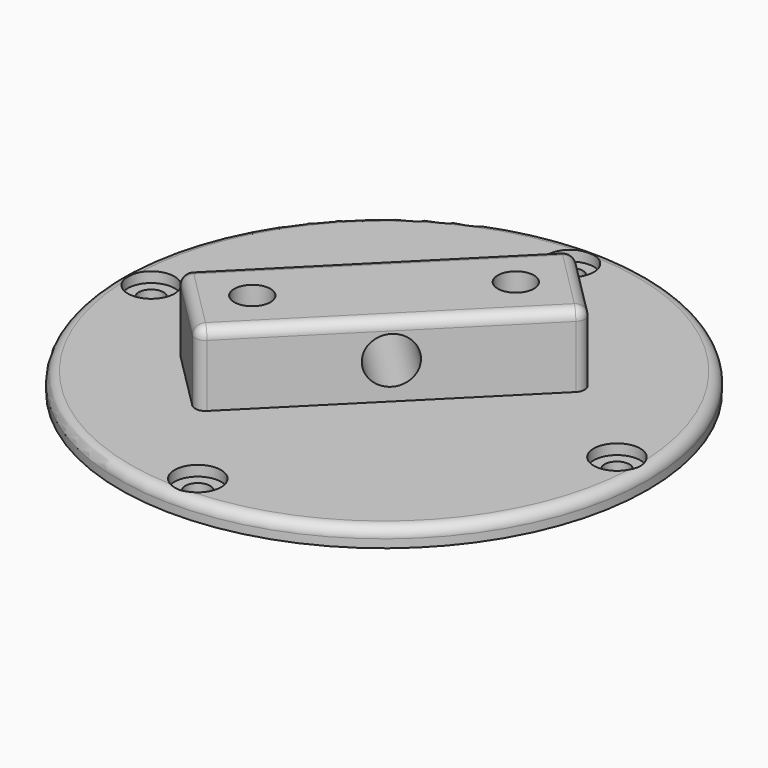
from build123d import *

# Parameters (mm, degrees)
F0_R         = 25.5
F0_R_2       = 1.2
F1_DEPTH     = 1.8
F2_R         = 2.25
F3_DEPTH     = 1
F4_R         = 1.75
F5_DEPTH     = 7
F6_START     = 2
F6_DEPTH     = 3
F7_R         = 2.25
F8_DEPTH     = 41.0634458405
F9_T1_DEPTH  = 6
F9_T3_DEPTH  = 8
F9_T5_DEPTH  = 28
F9_T7_DEPTH  = 28
F9_T9_DEPTH  = 8
F9_S13_W     = 1
F9_S13_H     = 1
F9_T14_DEPTH = 1
F9_T20_DEPTH = 1
F9_S25_W     = 1
F9_S25_H     = 1
F9_T26_DEPTH = 1
F9_T32_DEPTH = 1


# Not quite as in the source:
# - a fillet or chamfer that OpenCascade refuses, or shapes differently, is made with other operations: its cross-section is extruded or revolved along the edge and cut away or added


with BuildPart() as f1:
    # F0 (on Top) → F1 (new body)
    with BuildSketch(Plane.XY):
        Circle(F0_R)
        with Locations((0, -22.5)):
            Circle(F0_R_2, mode=Mode.SUBTRACT)
        with Locations((-22.5, 0)):
            Circle(F0_R_2, mode=Mode.SUBTRACT)
        with Locations((22.5, 0)):
            Circle(F0_R_2, mode=Mode.SUBTRACT)
        with Locations((0, 22.5)):
            Circle(F0_R_2, mode=Mode.SUBTRACT)
    extrude(amount=F1_DEPTH)

    # F2 (on face) → F3 (cut)
    with BuildSketch(Plane.XY.offset(1.8)):
        with Locations((0, -22.5)):
            Circle(F2_R)
        with Locations((-22.5, 0)):
            Circle(F2_R)
        with Locations((0, 22.5)):
            Circle(F2_R)
        with Locations((22.5, 0)):
            Circle(F2_R)
    extrude(amount=-F3_DEPTH, mode=Mode.SUBTRACT)

    # F4 (on face) → F5 (join)
    with BuildSketch(Plane.XY.offset(1.8)):
        Polygon((7.0710678119, 14.1421356237), (-14.1421356237, -7.0710678119), (-7.0710678119, -14.1421356237), (14.1421356237, 7.0710678119), align=None)
        Polygon((-6.1744923397, -10.4171330268), (-9.5205575546, -9.5205575546), (-10.4171330268, -6.1744923397), (-7.967643284, -3.7250025969), (-4.6215780691, -4.6215780691), (-3.7250025969, -7.967643284), align=None, mode=Mode.SUBTRACT)
        Polygon((3.7250025969, 7.967643284), (6.1744923397, 10.4171330268), (9.5205575546, 9.5205575546), (10.4171330268, 6.1744923397), (7.967643284, 3.7250025969), (4.6215780691, 4.6215780691), align=None, mode=Mode.SUBTRACT)
        Polygon((-10.4171330268, -6.1744923397), (-9.5205575546, -9.5205575546), (-6.1744923397, -10.4171330268), (-3.7250025969, -7.967643284), (-4.6215780691, -4.6215780691), (-7.967643284, -3.7250025969), align=None)
        with Locations((-7.0710678119, -7.0710678119)):
            Circle(F4_R, mode=Mode.SUBTRACT)
        Polygon((9.5205575546, 9.5205575546), (6.1744923397, 10.4171330268), (3.7250025969, 7.967643284), (4.6215780691, 4.6215780691), (7.967643284, 3.7250025969), (10.4171330268, 6.1744923397), align=None)
        with Locations((7.0710678119, 7.0710678119)):
            Circle(F4_R, mode=Mode.SUBTRACT)
    extrude(amount=F5_DEPTH)

    # F4 (on face) → F6 (cut)
    with BuildSketch(Plane.XY.offset(1.8).offset(F6_START)):
        Polygon((-10.4171330268, -6.1744923397), (-9.5205575546, -9.5205575546), (-6.1744923397, -10.4171330268), (-3.7250025969, -7.967643284), (-4.6215780691, -4.6215780691), (-7.967643284, -3.7250025969), align=None)
        with Locations((-7.0710678119, -7.0710678119)):
            Circle(F4_R, mode=Mode.SUBTRACT)
        Polygon((9.5205575546, 9.5205575546), (6.1744923397, 10.4171330268), (3.7250025969, 7.967643284), (4.6215780691, 4.6215780691), (7.967643284, 3.7250025969), (10.4171330268, 6.1744923397), align=None)
        with Locations((7.0710678119, 7.0710678119)):
            Circle(F4_R, mode=Mode.SUBTRACT)
    extrude(amount=F6_DEPTH, mode=Mode.SUBTRACT)

    # F7 (on face) → F8 (cut, through all)
    with BuildSketch(Plane(origin=(-3.5355339059, 3.5355339059, 0), x_dir=(-0.7071067812, -0.7071067812, 0), z_dir=(-0.7071067812, 0.7071067812, 0))):
        with Locations((0, 5.3)):
            Circle(F7_R)
    extrude(amount=-F8_DEPTH, mode=Mode.SUBTRACT)

    # F9: fillet of radius 1 on 9 edges, made by hand

    # F9_s2 → F9_t1 (cut)
    with BuildSketch(Plane.XY.offset(1.8)):
        with BuildLine():
            ThreePointArc((-13.4350288425, -6.3639610307), (-13.7279220614, -7.0710678119), (-13.4350288425, -7.7781745931))
            Line((-13.4350288425, -7.7781745931), (-14.1421356237, -7.0710678119))
            Line((-14.1421356237, -7.0710678119), (-13.4350288425, -6.3639610307))
        make_face()
        with BuildLine():
            ThreePointArc((-7.7781745931, -13.4350288425), (-7.0710678119, -13.7279220614), (-6.3639610307, -13.4350288425))
            Line((-6.3639610307, -13.4350288425), (-7.0710678119, -14.1421356237))
            Line((-7.0710678119, -14.1421356237), (-7.7781745931, -13.4350288425))
        make_face()
        with BuildLine():
            ThreePointArc((13.4350288425, 6.3639610307), (13.7279220614, 7.0710678119), (13.4350288425, 7.7781745931))
            Line((13.4350288425, 7.7781745931), (14.1421356237, 7.0710678119))
            Line((14.1421356237, 7.0710678119), (13.4350288425, 6.3639610307))
        make_face()
        with BuildLine():
            ThreePointArc((6.3639610307, 13.4350288425), (7.0710678119, 13.7279220614), (7.7781745931, 13.4350288425))
            Line((7.7781745931, 13.4350288425), (7.0710678119, 14.1421356237))
            Line((7.0710678119, 14.1421356237), (6.3639610307, 13.4350288425))
        make_face()
    extrude(amount=F9_T1_DEPTH, mode=Mode.SUBTRACT)

    # F9_s4 → F9_t3 (cut)
    with BuildSketch(Plane(origin=(-2.8284271247, 2.8284271247, 0), x_dir=(0, 0, 1), z_dir=(0.7071067812, -0.7071067812, 0))):
        with BuildLine():
            ThreePointArc((7.8, 15), (8.5071067812, 14.7071067812), (8.8, 14))
            Line((8.8, 14), (8.8, 15))
            Line((8.8, 15), (7.8, 15))
        make_face()
    extrude(amount=F9_T3_DEPTH, mode=Mode.SUBTRACT)

    # F9_s6 → F9_t5 (cut)
    with BuildSketch(Plane(origin=(9.8994949366, 9.8994949366, 0), x_dir=(0, 0, 1), z_dir=(-0.7071067812, -0.7071067812, 0))):
        with BuildLine():
            ThreePointArc((7.8, 5), (8.5071067812, 4.7071067812), (8.8, 4))
            Line((8.8, 4), (8.8, 5))
            Line((8.8, 5), (7.8, 5))
        make_face()
    extrude(amount=F9_T5_DEPTH, mode=Mode.SUBTRACT)

    # F9_s8 → F9_t7 (cut)
    with BuildSketch(Plane(origin=(-9.8994949366, -9.8994949366, 0), x_dir=(0, 0, 1), z_dir=(0.7071067812, 0.7071067812, 0))):
        with BuildLine():
            ThreePointArc((7.8, 5), (8.5071067812, 4.7071067812), (8.8, 4))
            Line((8.8, 4), (8.8, 5))
            Line((8.8, 5), (7.8, 5))
        make_face()
    extrude(amount=F9_T7_DEPTH, mode=Mode.SUBTRACT)

    # F9_s10 → F9_t9 (cut)
    with BuildSketch(Plane(origin=(2.8284271247, -2.8284271247, 0), x_dir=(0, 0, 1), z_dir=(-0.7071067812, 0.7071067812, 0))):
        with BuildLine():
            ThreePointArc((7.8, 15), (8.5071067812, 14.7071067812), (8.8, 14))
            Line((8.8, 14), (8.8, 15))
            Line((8.8, 15), (7.8, 15))
        make_face()
    extrude(amount=F9_T9_DEPTH, mode=Mode.SUBTRACT)


with BuildPart() as f9_tool12:
    # F9_s13 → F9_t14 (new body)
    with BuildSketch(Plane(origin=(-2.8284271247, 2.8284271247, 0), x_dir=(0, 0, 1), z_dir=(-0.7071067812, 0.7071067812, 0))):
        with Locations((8.3, -14.5)):
            Rectangle(F9_S13_W, F9_S13_H)
    extrude(amount=F9_T14_DEPTH)

    # F9_s15 → F9_t16 (revolve, cut)
    with BuildSketch(Plane(origin=(-12.7279220614, -7.0710678119, 7.8), x_dir=(0.5, 0.5, -0.7071067812), z_dir=(0.5, 0.5, 0.7071067812))):
        with BuildLine():
            ThreePointArc((0, -1), (1, 0), (0, 1))
            Line((0, 1), (0, -1))
        make_face()
    revolve(axis=Axis((-12.7279220614, -7.0710678119, 7.8), (-0.7071067812, 0.7071067812, 0)), mode=Mode.SUBTRACT)


with BuildPart() as f1_1:
    add(f1.part)

    # F9_t11: cut F9_tool12
    add(f9_tool12.part, mode=Mode.SUBTRACT)


with BuildPart() as f9_tool18:
    # F9_s19 → F9_t20 (new body)
    with BuildSketch(Plane.XY.offset(7.8)):
        Polygon((-7.0710678119, -12.7279220614), (-7.7781745931, -13.4350288425), (-7.0710678119, -14.1421356237), (-6.3639610307, -13.4350288425), align=None)
    extrude(amount=F9_T20_DEPTH)

    # F9_s21 → F9_t22 (revolve, cut)
    with BuildSketch(Plane(origin=(-7.0710678119, -12.7279220614, 7.8), x_dir=(0, 1, 0), z_dir=(1, 0, 0))):
        with BuildLine():
            ThreePointArc((0, -1), (1, 0), (0, 1))
            Line((0, 1), (0, -1))
        make_face()
    revolve(axis=Axis((-7.0710678119, -12.7279220614, 7.8), (0, 0, 1)), mode=Mode.SUBTRACT)


with BuildPart() as f1_2:
    add(f1_1.part)

    # F9_t17: cut F9_tool18
    add(f9_tool18.part, mode=Mode.SUBTRACT)


with BuildPart() as f9_tool24:
    # F9_s25 → F9_t26 (new body)
    with BuildSketch(Plane(origin=(-2.8284271247, 2.8284271247, 0), x_dir=(0, 0, 1), z_dir=(-0.7071067812, 0.7071067812, 0))):
        with Locations((8.3, 14.5)):
            Rectangle(F9_S25_W, F9_S25_H)
    extrude(amount=F9_T26_DEPTH)

    # F9_s27 → F9_t28 (revolve, cut)
    with BuildSketch(Plane(origin=(7.0710678119, 12.7279220614, 7.8), x_dir=(-0.5, -0.5, -0.7071067812), z_dir=(0.5, 0.5, -0.7071067812))):
        with BuildLine():
            ThreePointArc((0, -1), (1, 0), (0, 1))
            Line((0, 1), (0, -1))
        make_face()
    revolve(axis=Axis((7.0710678119, 12.7279220614, 7.8), (-0.7071067812, 0.7071067812, 0)), mode=Mode.SUBTRACT)


with BuildPart() as f1_3:
    add(f1_2.part)

    # F9_t23: cut F9_tool24
    add(f9_tool24.part, mode=Mode.SUBTRACT)


with BuildPart() as f9_tool30:
    # F9_s31 → F9_t32 (new body)
    with BuildSketch(Plane.XY.offset(7.8)):
        Polygon((12.7279220614, 7.0710678119), (13.4350288425, 6.3639610307), (14.1421356237, 7.0710678119), (13.4350288425, 7.7781745931), align=None)
    extrude(amount=F9_T32_DEPTH)

    # F9_s33 → F9_t34 (revolve, cut)
    with BuildSketch(Plane(origin=(12.7279220614, 7.0710678119, 7.8), x_dir=(-1, 0, 0), z_dir=(0, 1, 0))):
        with BuildLine():
            ThreePointArc((0, -1), (1, 0), (0, 1))
            Line((0, 1), (0, -1))
        make_face()
    revolve(axis=Axis((12.7279220614, 7.0710678119, 7.8), (0, 0, 1)), mode=Mode.SUBTRACT)


with BuildPart() as f1_4:
    add(f1_3.part)

    # F9_t29: cut F9_tool30
    add(f9_tool30.part, mode=Mode.SUBTRACT)

    # F9_s35 → F9_t36 (revolve, cut)
    with BuildSketch(Plane.XZ):
        with BuildLine():
            ThreePointArc((25.5, 0.8), (25.2071067812, 1.5071067812), (24.5, 1.8))
            Line((24.5, 1.8), (25.5, 1.8))
            Line((25.5, 1.8), (25.5, 0.8))
        make_face()
    revolve(axis=Axis((0, 0, 1.8), (0, 0, 1)), mode=Mode.SUBTRACT)


solid = f1_4.part
